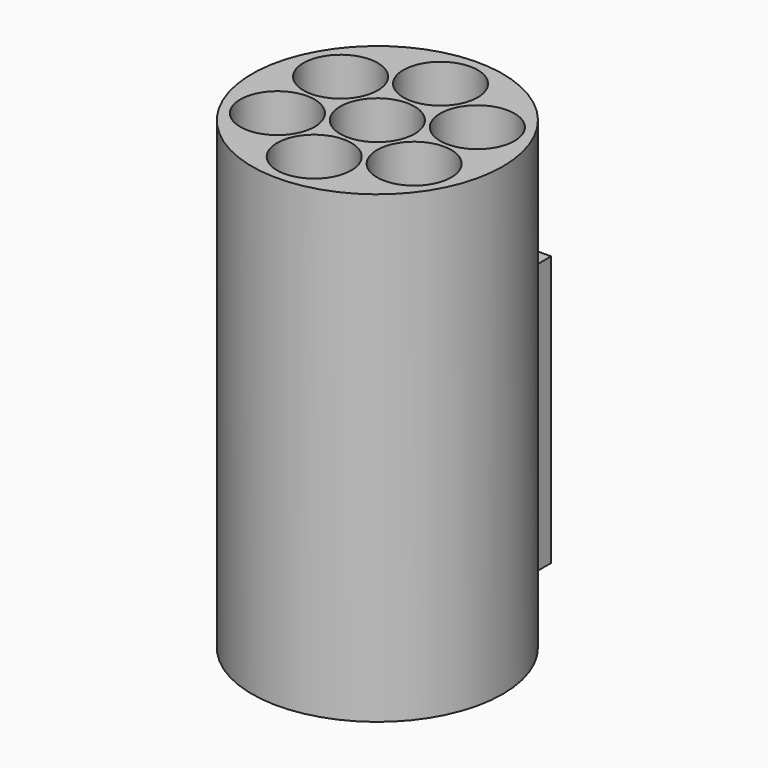
from build123d import *

# Parameters (mm, degrees)
F2_R         = 1.35
F3_DEPTH     = 5
F1_R         = 0.4
F4_DEPTH     = 5.001
F9_TEXT_SIZE = 4.0725106373
F10_DEPTH    = 0.35


# Not quite as in the source:
# - Text() gives the source's letters only with a copy of the font that has no kerning and outlines rounded to 1/6400 em; it was checked with that copy


with BuildPart() as f3:
    # F2 (on Top) → F3 (new body)
    with BuildSketch(Plane.XY):
        Circle(F2_R)
    extrude(amount=F3_DEPTH)

    # F1 (on Top) → F4 (cut, through all)
    with BuildSketch(Plane.XY):
        Circle(F1_R)
        with Locations((0, 0.85)):
            Circle(F1_R)
        with Locations((0.7361215932, 0.425)):
            Circle(F1_R)
        with Locations((0.7361215932, -0.425)):
            Circle(F1_R)
        with Locations((0, -0.85)):
            Circle(F1_R)
        with Locations((-0.7361215932, -0.425)):
            Circle(F1_R)
        with Locations((-0.7361215932, 0.425)):
            Circle(F1_R)
    extrude(amount=F4_DEPTH, mode=Mode.SUBTRACT)

    # F9 (on face) → F10 (join)
    with BuildSketch(Plane(origin=(0, 1.05, 0), x_dir=(-1, 0, 0), z_dir=(0, 1, 0))):
        with Locations((-1.1491243131, 0.4769489169)):
            Text('II', F9_TEXT_SIZE, font='Open Sans', text_align=(TextAlign.LEFT, TextAlign.BOTTOM))
    extrude(amount=F10_DEPTH)


solid = f3.part
